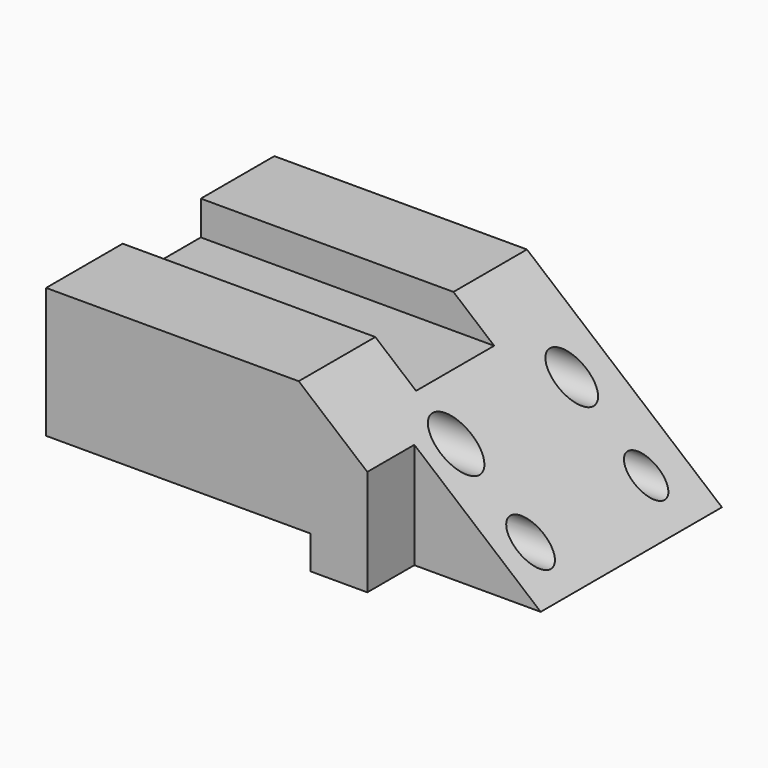
from build123d import *

# Parameters (mm, degrees)
F0_W        = 114.5921349525
F0_H        = 72.0440149307
F1_DEPTH    = 41.3016155362
F2_W        = 66.8072551489
F2_H        = 8.4119299427
F6_DEPTH    = 72.0450149307
F7_T1_DEPTH = 333.9084750306
F3_W        = 31.901553337
F3_H        = 14.8452445865
F4_DEPTH    = 41.3026155362
F5_W        = 24.6558189392
F5_H        = 8.6286962032
F8_DEPTH    = 113.0144836478
F9_R        = 4.6345272192
F9_R_2      = 4.97207371
F10_DEPTH   = 113.0144836478


# Not quite as in the source:
# - a fillet or chamfer that OpenCascade refuses, or shapes differently, is made with other operations: its cross-section is extruded or revolved along the edge and cut away or added


with BuildPart() as f1:
    # F0 (on Top) → F1 (new body)
    with BuildSketch(Plane.XY):
        Rectangle(F0_W, F0_H)
    extrude(amount=F1_DEPTH)

    # F2 (on face) → F6 (cut, through all)
    with BuildSketch(Plane.XZ.offset(36.0220074654)):
        with Locations((-23.8924399018, 4.2059649713)):
            Rectangle(F2_W, F2_H)
    extrude(amount=-F6_DEPTH, mode=Mode.SUBTRACT)

    # F7: chamfer of 50.8 x 42.6262612638 on 1 edges, made by hand

    # F7_s2 → F7_t1 (cut)
    with BuildSketch(Plane.XZ.offset(-166.9542375153)):
        Polygon((57.2960674763, -1.3246457276), (6.4960674763, 41.3016155362), (57.2960674763, 41.3016155362), align=None)
    extrude(amount=F7_T1_DEPTH, mode=Mode.SUBTRACT)

    # F3 (on face) → F4 (cut, through all)
    with BuildSketch(Plane(origin=(0, 0, 0), x_dir=(1, 0, 0), z_dir=(0, 0, -1))):
        with Locations((39.766639503, 28.5993851721)):
            Rectangle(F3_W, F3_H)
    extrude(amount=-F4_DEPTH, mode=Mode.SUBTRACT)

    # F5 (on face) → F8 (cut, through all)
    with BuildSketch(Plane(origin=(-57.2960674763, 0, 0), x_dir=(0, -1, 0), z_dir=(-1, 0, 0))):
        with Locations((-0.4837103188, 36.9872674346)):
            Rectangle(F5_W, F5_H)
    extrude(amount=-F8_DEPTH, mode=Mode.SUBTRACT)

    # F9 (on face) → F10 (cut, through all)
    with BuildSketch(Plane(origin=(-57.2960674763, 0, 0), x_dir=(0, -1, 0), z_dir=(-1, 0, 0))):
        with Locations((-24.6397461742, 24.1792052984)):
            Circle(F9_R)
        with Locations((11.8441991508, 24.1792052984)):
            Circle(F9_R_2)
        with BuildLine():
            ThreePointArc((16.128482923, 8.4119299427), (11.8441991508, 12.6962137149), (7.5599153786, 8.4119299427))
            Line((7.5599153786, 8.4119299427), (16.128482923, 8.4119299427))
        make_face()
        with BuildLine():
            ThreePointArc((-28.5501872317, 8.4119299427), (-24.6397461742, 4.5014888852), (-20.7293051168, 8.4119299427))
            Line((-20.7293051168, 8.4119299427), (-28.5501872317, 8.4119299427))
        make_face()
        with BuildLine():
            Line((-28.5501872317, 8.4119299427), (-20.7293051168, 8.4119299427))
            ThreePointArc((-20.7293051168, 8.4119299427), (-24.6397461742, 12.3223710001), (-28.5501872317, 8.4119299427))
        make_face()
        with BuildLine():
            Line((16.128482923, 8.4119299427), (7.5599153786, 8.4119299427))
            ThreePointArc((7.5599153786, 8.4119299427), (11.8441991508, 4.1276461705), (16.128482923, 8.4119299427))
        make_face()
    extrude(amount=-F10_DEPTH, mode=Mode.SUBTRACT)


solid = f1.part
